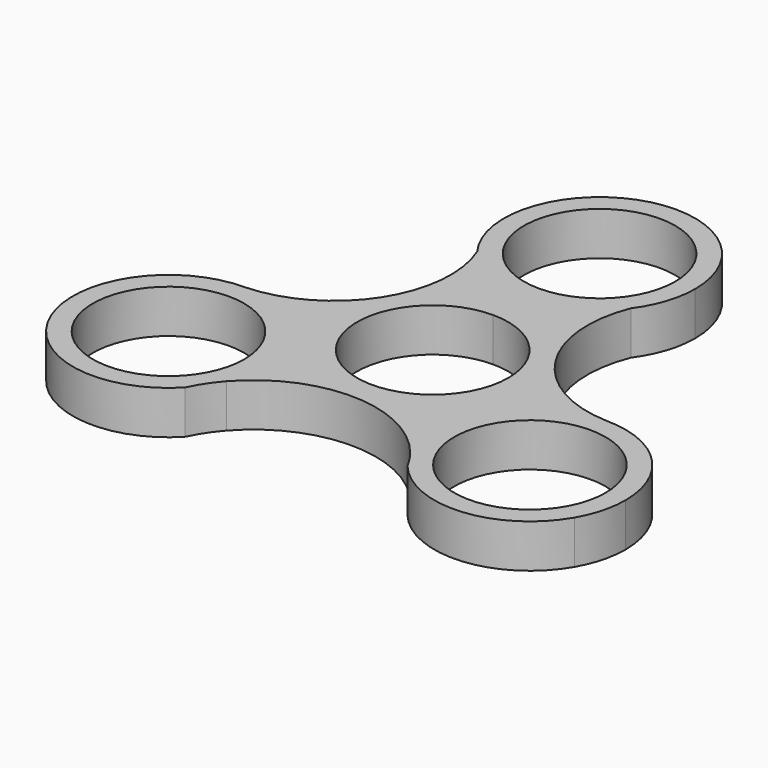
from build123d import *

# Parameters (mm, degrees)
F1_R     = 11.049
F2_DEPTH = 6.35
F4_DEPTH = 6.35
F0_R     = 44.45
F0_R_2   = 11.049
F5_DEPTH = 113
F7_DEPTH = 6.351


# Not quite as in the source:
# - an extrude ends at something that could not be found from the text; its depth is read off the source's solid


with BuildPart() as f2:
    # F1 (on face) → F2 (new body)
    with BuildSketch(Plane.XY):
        with BuildLine():
            ThreePointArc((11.2333605356, 22.1750309406), (6.2904881464, 18.0064015264), (0, 16.51))
            ThreePointArc((0, 16.51), (-6.2904881464, 18.0064015264), (-11.2333605356, 22.1750309406))
            ThreePointArc((-11.2333605356, 22.1750309406), (-12.7087939307, 6.5033813584), (-26.3964543073, -1.27))
            ThreePointArc((-26.3964543073, -1.27), (-16.5181725742, -5.3617182668), (-12.4264543073, -15.24))
            ThreePointArc((-12.4264543073, -15.24), (-12.7102714474, -18.0416599946), (-13.5501907032, -20.7294818894))
            ThreePointArc((-13.5501907032, -20.7294818894), (0.3483634498, -14.677920264), (13.8964774264, -21.477906538))
            ThreePointArc((13.8964774264, -21.477906538), (14.5157040294, -7.8909406838), (26.3964543073, -1.27))
            ThreePointArc((26.3964543073, -1.27), (12.7154911257, 6.507712775), (11.2333605356, 22.1750309406))
        make_face()
        with BuildLine():
            ThreePointArc((0, 13.97), (9.8782817332, 9.8782817332), (13.97, 0))
            ThreePointArc((13.97, 0), (-9.8782817332, -9.8782817332), (0, 13.97))
        make_face(mode=Mode.SUBTRACT)
        with BuildLine():
            ThreePointArc((-11.2333605356, 22.1750309406), (-6.2904881464, 18.0064015264), (0, 16.51))
            ThreePointArc((0, 16.51), (6.2904881464, 18.0064015264), (11.2333605356, 22.1750309406))
            ThreePointArc((11.2333605356, 22.1750309406), (13.2682128918, 26.1078807588), (13.97, 30.48))
            ThreePointArc((13.97, 30.48), (9.8782817686, 40.3582816978), (1.001e-07, 44.45))
            ThreePointArc((1.001e-07, 44.45), (-12.473598451, 36.7704881911), (-11.2333605356, 22.1750309406))
        make_face()
        with BuildLine():
            ThreePointArc((11.049, 30.48), (7.8128228253, 22.6671771747), (0, 19.431))
            ThreePointArc((0, 19.431), (-7.8128228253, 38.2928228253), (11.049, 30.48))
        make_face(mode=Mode.SUBTRACT)
        with BuildLine():
            ThreePointArc((-12.4264543073, -15.24), (-16.5181725742, -5.3617182668), (-26.3964543073, -1.27))
            ThreePointArc((-26.3964543073, -1.27), (-38.4948290673, -8.2549997732), (-38.4948294602, -22.2249995463))
            ThreePointArc((-38.4948294602, -22.2249995463), (-28.0548757974, -29.11121257), (-16.2857729321, -24.8802812266))
            ThreePointArc((-16.2857729321, -24.8802812266), (-15.0629921605, -22.709312564), (-13.5501907032, -20.7294818894))
            ThreePointArc((-13.5501907032, -20.7294818894), (-12.7102714474, -18.0416599946), (-12.4264543073, -15.24))
        make_face()
        with Locations((-26.3964543073, -15.24)):
            Circle(F1_R, mode=Mode.SUBTRACT)
        with BuildLine():
            ThreePointArc((40.3664543073, -15.24), (36.2747360405, -5.3617182668), (26.3964543073, -1.27))
            ThreePointArc((26.3964543073, -1.27), (14.5157040294, -7.8909406838), (13.8964774264, -21.477906538))
            ThreePointArc((13.8964774264, -21.477906538), (14.8325747733, -22.7814148116), (15.6479806578, -24.1636323436))
            ThreePointArc((15.6479806578, -24.1636323436), (27.5776113359, -29.1599773015), (38.4948290898, -22.2250001877))
            ThreePointArc((38.4948290898, -22.2250001877), (39.8904380726, -18.8557021648), (40.3664543073, -15.24))
        make_face()
        with Locations((26.3964543073, -15.24)):
            Circle(F1_R, mode=Mode.SUBTRACT)
    extrude(amount=F2_DEPTH)

    # F3 (on face) → F4 (join)
    with BuildSketch(Plane.XY):
        with BuildLine():
            ThreePointArc((0, 13.97), (-9.8782817332, -9.8782817332), (13.97, 0))
            ThreePointArc((13.97, 0), (9.8782817332, 9.8782817332), (0, 13.97))
        make_face()
        with BuildLine():
            ThreePointArc((11.049, 0), (-7.8128228253, -7.8128228253), (0, 11.049))
            ThreePointArc((0, 11.049), (7.8128228253, 7.8128228253), (11.049, 0))
        make_face(mode=Mode.SUBTRACT)
    extrude(amount=F4_DEPTH)

    # F0 (on Top) → F5 (cut, through all)
    with BuildSketch(Plane.XY):
        Circle(F0_R)
        with Locations((-26.3964543073, -15.24)):
            Circle(F0_R_2, mode=Mode.SUBTRACT)
        with Locations((26.3964543073, -15.24)):
            Circle(F0_R_2, mode=Mode.SUBTRACT)
        with BuildLine():
            ThreePointArc((0, 11.049), (7.8128228253, 7.8128228253), (11.049, 0))
            ThreePointArc((11.049, 0), (-7.8128228253, -7.8128228253), (0, 11.049))
        make_face(mode=Mode.SUBTRACT)
        with BuildLine():
            ThreePointArc((11.049, 30.48), (7.8128228253, 22.6671771747), (0, 19.431))
            ThreePointArc((0, 19.431), (-7.8128228253, 38.2928228253), (11.049, 30.48))
        make_face(mode=Mode.SUBTRACT)
    extrude(amount=-F5_DEPTH, mode=Mode.SUBTRACT)

    # F6 (on face) → F7 (cut, through all)
    with BuildSketch(Plane.XY.offset(6.35)):
        with BuildLine():
            Line((-26.3964543073, 15.7554745193), (-26.3964543073, -1.27))
            ThreePointArc((-26.3964543073, -1.27), (-12.7087939307, 6.5033813584), (-11.2333605356, 22.1750309406))
            Line((-11.2333605356, 22.1750309406), (-26.3964543073, 15.7554745193))
        make_face()
    extrude(amount=-F7_DEPTH, mode=Mode.SUBTRACT)


solid = f2.part
